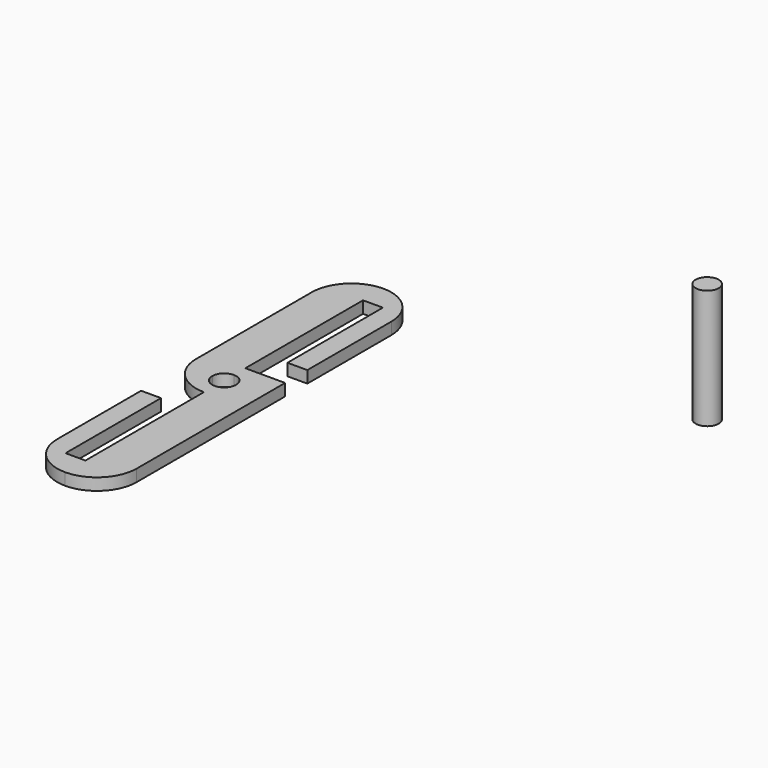
from build123d import *

# Parameters (mm, degrees)
F1_DEPTH = 1.5
F2_R     = 4.99999
F0_R     = 1.45
F3_DEPTH = 15


# Not quite as in the source:
# - a fillet or chamfer is up to 0.001 mm smaller than in the source, because OpenCascade refuses the exact size


with BuildPart() as f1:
    # F0 (on Top) → F1 (new body)
    with BuildSketch(Plane.XY):
        Polygon((2.5, 6.8097828329), (5, 6.8097828329), (5, 25), (-5, 25), (-5, 3.3164751772), (0, 3.3164751772), (0, 21.8097828329), (2.5, 21.8097828329), align=None)
        Polygon((-5, -25), (5, -25), (5, -3.1835248228), (0, -3.1835248228), (0, -21.8097828329), (-2.5, -21.8097828329), (-2.5, -6.8097828329), (-5, -6.8097828329), align=None)
        with BuildLine():
            Line((1.5, 0), (5, 0))
            Line((5, 0), (5, 3.3164751772))
            Line((5, 3.3164751772), (0, 3.3164751772))
            Line((0, 3.3164751772), (0, 1.5))
            ThreePointArc((0, 1.5), (1.0606601718, 1.0606601718), (1.5, 0))
        make_face()
        with BuildLine():
            Line((-5, 3.3164751772), (-5, 0))
            Line((-5, 0), (-1.5, 0))
            ThreePointArc((-1.5, 0), (-1.0606601718, 1.0606601718), (0, 1.5))
            Line((0, 1.5), (0, 3.3164751772))
            Line((0, 3.3164751772), (-5, 3.3164751772))
        make_face()
        with BuildLine():
            Line((-5, -3.1835248228), (0, -3.1835248228))
            Line((0, -3.1835248228), (0, -1.5))
            ThreePointArc((0, -1.5), (-1.0606601718, -1.0606601718), (-1.5, 0))
            Line((-1.5, 0), (-5, 0))
            Line((-5, 0), (-5, -3.1835248228))
        make_face()
        with BuildLine():
            Line((0, -3.1835248228), (5, -3.1835248228))
            Line((5, -3.1835248228), (5, 0))
            Line((5, 0), (1.5, 0))
            ThreePointArc((1.5, 0), (1.0606601718, -1.0606601718), (0, -1.5))
            Line((0, -1.5), (0, -3.1835248228))
        make_face()
    extrude(amount=-F1_DEPTH)

    # F2 (radius 5 in the source; OpenCascade refuses exactly that, so slightly less here)
    f2_edges = [f1.edges().sort_by_distance(p)[0] for p in [
        (5, 25, -0.75),
        (-5, 25, -0.75),
        (-5, -3.183525, -0.75),
        (5, -25, -0.75),
        (-5, -25, -0.75),
    ]]
    fillet(f2_edges, radius=F2_R)


with BuildPart() as f3:
    # F0 (on Top) → F3 (new body)
    with BuildSketch(Plane.XY):
        with Locations((42.2054678202, 23.1356341392)):
            Circle(F0_R)
    extrude(amount=F3_DEPTH)


solid = Compound([f1.part, f3.part])
